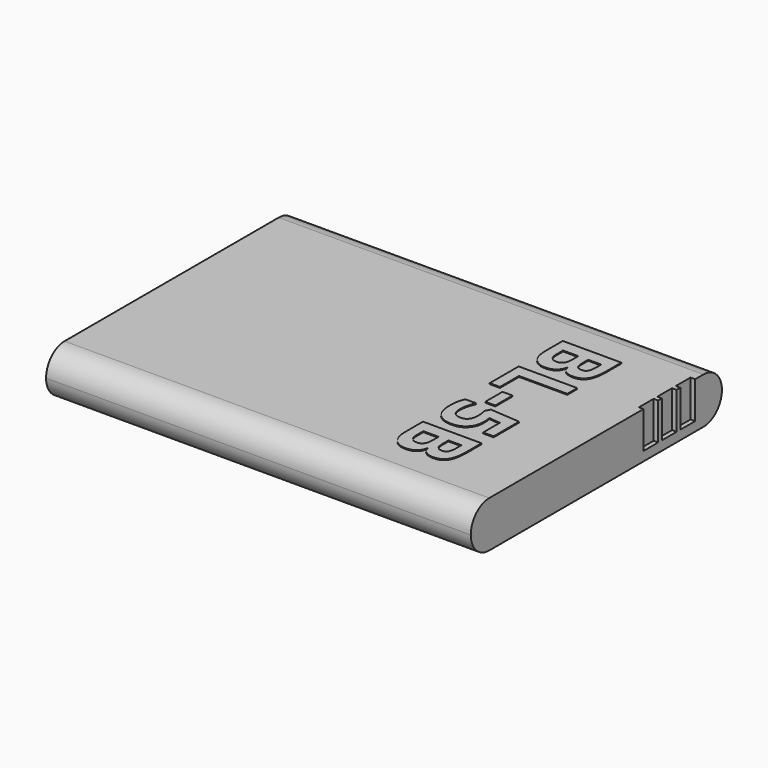
from build123d import *

# Parameters (mm, degrees)
F0_W         = 46
F0_H         = 34
F1_DEPTH     = 5
F2_R         = 2.49999
F3_W         = 2
F3_H         = 4
F4_DEPTH     = 0.5
F5_TEXT_SIZE = 8.8859269133
F6_DEPTH     = 0.1


# Not quite as in the source:
# - a fillet or chamfer is up to 0.001 mm smaller than in the source, because OpenCascade refuses the exact size
# - Text() gives the source's letters only with a copy of the font that has no kerning and outlines rounded to 1/6400 em; it was checked with that copy


with BuildPart() as f1:
    # F0 (on Top) → F1 (new body)
    with BuildSketch(Plane.XY):
        Rectangle(F0_W, F0_H)
    extrude(amount=F1_DEPTH)

    # F2 (radius 2.5 in the source; OpenCascade refuses exactly that, so slightly less here)
    f2_edges = [f1.edges().sort_by_distance(p)[0] for p in [
        (0, 17, 5),
        (0, 17, 0),
        (0, -17, 5),
        (0, -17, 0),
    ]]
    fillet(f2_edges, radius=F2_R)

    # F3 (on face) → F4 (cut)
    with BuildSketch(Plane.YZ.offset(23)):
        with Locations((12.3746041209, 3)):
            Rectangle(F3_W, F3_H)
        with Locations((9.8746041209, 3)):
            Rectangle(F3_W, F3_H)
        with Locations((7.3746041209, 3)):
            Rectangle(F3_W, F3_H)
    extrude(amount=-F4_DEPTH, mode=Mode.SUBTRACT)

    # F5 (on face) → F6 (join)
    with BuildSketch(Plane.XY.offset(5)):
        with Locations(Location((10, 12.5), (0, 0, -90))):
            Text('BL-5B', F5_TEXT_SIZE, font='Open Sans', font_style=FontStyle.BOLD, text_align=(TextAlign.LEFT, TextAlign.BOTTOM))
    extrude(amount=F6_DEPTH)


solid = f1.part
